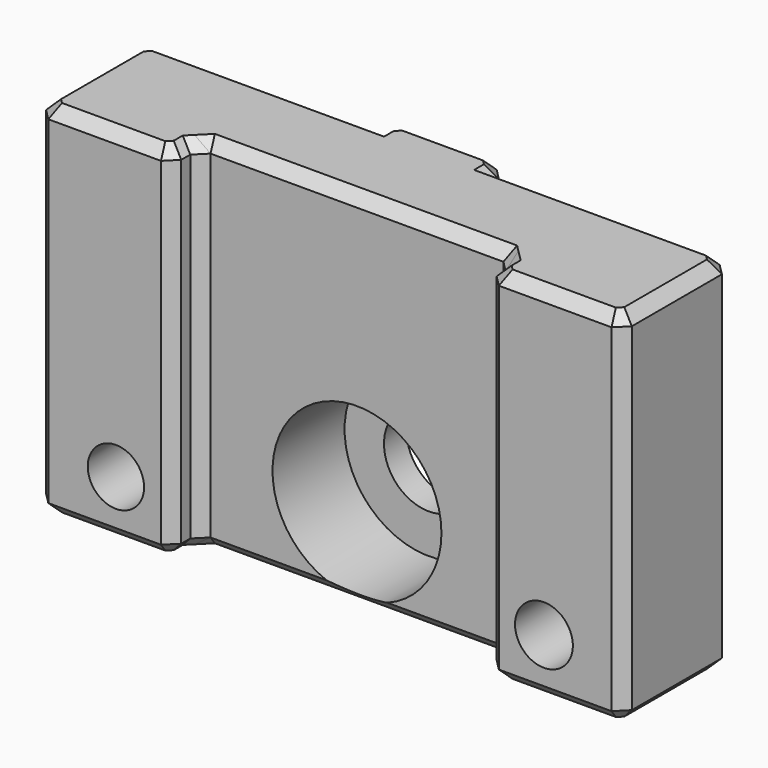
from build123d import *

# Parameters (mm, degrees)
F1_DEPTH      = 16
F3_R          = 1.25
F4_DEPTH      = 25
F5_R          = 2
F6_DEPTH      = 25
F5_R_2        = 3.75
F7_DEPTH      = 4
F8_SIZE       = 0.49999
F9_T1_DEPTH   = 3.278775627
F9_T3_DEPTH   = 7.571702988
F9_T5_DEPTH   = 3.278775627
F9_T7_DEPTH   = 6.571702988
F9_T9_DEPTH   = 7.571702988
F9_T11_DEPTH  = 3.278775627
F9_T13_DEPTH  = 3.278775627
F9_T15_DEPTH  = 3.278775627
F9_T17_DEPTH  = 7.571702988
F9_T19_DEPTH  = 3.278775627
F9_T24_DEPTH  = 12.571692988
F9_T29_DEPTH  = 2.821692988
F9_T34_DEPTH  = 3.278775627
F9_T39_DEPTH  = 3.278775627
F9_T44_DEPTH  = 2.821692988
F9_T49_DEPTH  = 3.071702988
F9_T54_DEPTH  = 12.571692988
F9_T59_DEPTH  = 3.278775627
F9_T65_DEPTH  = 15.571702988
F9_T71_DEPTH  = 3.278775627
F9_T77_DEPTH  = 3.071702988
F9_T82_DEPTH  = 12.571692988
F9_T87_DEPTH  = 2.821692988
F9_T92_DEPTH  = 3.278775627
F9_T97_DEPTH  = 3.278775627
F9_T102_DEPTH = 2.821692988
F9_T107_DEPTH = 3.071702988
F9_T112_DEPTH = 12.571692988
F9_T117_DEPTH = 3.278775627
F9_T123_DEPTH = 15.571702988
F9_T129_DEPTH = 3.278775627
F9_T135_DEPTH = 3.071702988


# Not quite as in the source:
# - a fillet or chamfer that OpenCascade refuses, or shapes differently, is made with other operations: its cross-section is extruded or revolved along the edge and cut away or added
# - a fillet or chamfer is up to 0.001 mm smaller than in the source, because OpenCascade refuses the exact size


with BuildPart() as f1:
    # F0 (on Top) → F1 (new body)
    with BuildSketch(Plane.XY):
        Polygon((-2.5, 3.4985319469), (-13, 3.4985319469), (-13, -2.5014680531), (-7, -2.5014680531), (-7, -1.0014680531), (7, -1.0014680531), (7, -2.5014680531), (13, -2.5014680531), (13, 3.4985319469), (2.5, 3.4985319469), (2.5, 4.2485319469), (-2.5, 4.2485319469), align=None)
    extrude(amount=F1_DEPTH)

    # F3 (on offset) → F4 (cut)
    with BuildSketch(Plane.XZ.offset(2.5014680531)):
        with Locations((-9.5, 2.5)):
            Circle(F3_R)
        with BuildLine():
            ThreePointArc((10.7833518404, 2.5), (9.5, 3.7833518404), (8.2166481596, 2.5))
            ThreePointArc((8.2166481596, 2.5), (9.5, 1.2166481596), (10.7833518404, 2.5))
        make_face()
    extrude(amount=-F4_DEPTH, mode=Mode.SUBTRACT)

    # F5 (on face) → F6 (cut)
    with BuildSketch(Plane.XZ.offset(1.0014680531)):
        with Locations((0, 4)):
            Circle(F5_R)
    extrude(amount=-F6_DEPTH, mode=Mode.SUBTRACT)

    # F5 (on face) → F7 (cut)
    with BuildSketch(Plane.XZ.offset(1.0014680531)):
        with Locations((0, 4)):
            Circle(F5_R_2)
        with Locations((0, 4)):
            Circle(F5_R, mode=Mode.SUBTRACT)
    extrude(amount=-F7_DEPTH, mode=Mode.SUBTRACT)

    # F8 (size 0.5 in the source; OpenCascade refuses exactly that, so slightly less here)
    f8_edges = [f1.edges().sort_by_distance(p)[0] for p in [
        (-2.5, 4.248532, 8),
        (2.5, 4.248532, 8),
        (13, 3.498532, 8),
        (-13, 3.498532, 8),
        (-13, -2.501468, 8),
        (7, -2.501468, 8),
        (13, -2.501468, 8),
        (-7, -2.501468, 8),
        (-7, -1.001468, 8),
        (7, -1.001468, 8),
    ]]
    chamfer(f8_edges, length=F8_SIZE)

    # F9: chamfer of 0.5 on 44 edges, made by hand

    # F9_s2 → F9_t1 (cut)
    with BuildSketch(Plane(origin=(3.5915117866, -3.5915117866, 0), x_dir=(0, 0, 1), z_dir=(0.7071067812, -0.7071067812, 0))):
        Polygon((15.5, -11.3126774998), (16, -10.8126774998), (16, -11.3126774998), align=None)
        Polygon((0, -10.8126774998), (0.5, -11.3126774998), (0, -11.3126774998), align=None)
    extrude(amount=F9_T1_DEPTH, mode=Mode.SUBTRACT)

    # F9_s4 → F9_t3 (cut)
    with BuildSketch(Plane.XZ.offset(-4.2843834409)):
        Polygon((12.5, 16), (13, 15.5), (13, 16), align=None)
        Polygon((-12.5, 16), (-13, 15.5), (-13, 16), align=None)
        Polygon((12.5, 0), (13, 0.5), (13, 0), align=None)
        Polygon((-12.5, 0), (-13, 0.5), (-13, 0), align=None)
    extrude(amount=F9_T3_DEPTH, mode=Mode.SUBTRACT)

    # F9_s6 → F9_t5 (cut)
    with BuildSketch(Plane(origin=(6.4084882134, 6.4084882134, 0), x_dir=(0, 0, 1), z_dir=(-0.7071067812, -0.7071067812, 0))):
        Polygon((16, -10.1076468592), (15.5, -10.6076468592), (16, -10.6076468592), align=None)
        Polygon((0, -10.1076468592), (0.5, -10.6076468592), (0, -10.6076468592), align=None)
    extrude(amount=F9_T5_DEPTH, mode=Mode.SUBTRACT)

    # F9_s8 → F9_t7 (cut)
    with BuildSketch(Plane.YZ.offset(-3.285851494)):
        Polygon((3.7485319469, 16), (4.2485319469, 15.5), (4.2485319469, 16), align=None)
        Polygon((3.7485319469, 0), (4.2485319469, 0.5), (4.2485319469, 0), align=None)
    extrude(amount=F9_T7_DEPTH, mode=Mode.SUBTRACT)

    # F9_s10 → F9_t9 (cut)
    with BuildSketch(Plane.YZ.offset(6.214148506)):
        Polygon((-2.0014680531, 16), (-2.5014680531, 15.5), (-2.5014680531, 16), align=None)
        Polygon((-2.0014680531, 0), (-2.5014680531, 0.5), (-2.5014680531, 0), align=None)
    extrude(amount=F9_T9_DEPTH, mode=Mode.SUBTRACT)

    # F9_s12 → F9_t11 (cut)
    with BuildSketch(Plane(origin=(5.9099562665, -5.9099562665, 0), x_dir=(0, 0, 1), z_dir=(-0.7071067812, 0.7071067812, 0))):
        Polygon((16, 4.0344887646), (15.5, 3.5344887646), (16, 3.5344887646), align=None)
        Polygon((0, 4.0344887646), (0.5, 3.5344887646), (0, 3.5344887646), align=None)
    extrude(amount=F9_T11_DEPTH, mode=Mode.SUBTRACT)

    # F9_s14 → F9_t13 (cut)
    with BuildSketch(Plane(origin=(-3.5915117866, -3.5915117866, 0), x_dir=(0, 0, 1), z_dir=(-0.7071067812, -0.7071067812, 0))):
        Polygon((16, 10.8126774998), (15.5, 11.3126774998), (16, 11.3126774998), align=None)
        Polygon((0, 10.8126774998), (0.5, 11.3126774998), (0, 11.3126774998), align=None)
    extrude(amount=F9_T13_DEPTH, mode=Mode.SUBTRACT)

    # F9_s16 → F9_t15 (cut)
    with BuildSketch(Plane(origin=(-6.4084882134, 6.4084882134, 0), x_dir=(0, 0, 1), z_dir=(0.7071067812, -0.7071067812, 0))):
        Polygon((16, 10.1076468592), (15.5, 10.6076468592), (16, 10.6076468592), align=None)
        Polygon((0, 10.1076468592), (0.5, 10.6076468592), (0, 10.6076468592), align=None)
    extrude(amount=F9_T15_DEPTH, mode=Mode.SUBTRACT)

    # F9_s18 → F9_t17 (cut)
    with BuildSketch(Plane.YZ.offset(-13.785851494)):
        Polygon((-2.0014680531, 16), (-2.5014680531, 15.5), (-2.5014680531, 16), align=None)
        Polygon((-2.0014680531, 0), (-2.5014680531, 0.5), (-2.5014680531, 0), align=None)
    extrude(amount=F9_T17_DEPTH, mode=Mode.SUBTRACT)

    # F9_s20 → F9_t19 (cut)
    with BuildSketch(Plane(origin=(-5.9099562665, -5.9099562665, 0), x_dir=(0, 0, 1), z_dir=(0.7071067812, 0.7071067812, 0))):
        Polygon((16, -4.0344887646), (15.5, -3.5344887646), (16, -3.5344887646), align=None)
        Polygon((0, -4.0344887646), (0.5, -3.5344887646), (0, -3.5344887646), align=None)
    extrude(amount=F9_T19_DEPTH, mode=Mode.SUBTRACT)


with BuildPart() as f9_tool22:
    # F9_s23 → F9_t24 (new body)
    with BuildSketch(Plane.YZ.offset(13.785851494)):
        Polygon((3.4985319469, 15.5), (2.9985319469, 16), (3.4985319469, 16), align=None)
    extrude(amount=-F9_T24_DEPTH)

    split(bisect_by=Plane(origin=(9, 0, 9), x_dir=(0, 1, 0), z_dir=(0.7071067812, 0, 0.7071067812)), keep=Keep.TOP)


with BuildPart() as f1_1:
    add(f1.part)

    # F9_t21: cut F9_tool22
    add(f9_tool22.part, mode=Mode.SUBTRACT)


with BuildPart() as f9_tool27:
    # F9_s28 → F9_t29 (new body)
    with BuildSketch(Plane.XZ.offset(-2.2126904529)):
        Polygon((2.5, 15.5), (2, 16), (2.5, 16), align=None)
    extrude(amount=-F9_T29_DEPTH)

    split(bisect_by=Plane(origin=(0, 9.4992659735, 9.4992659735), x_dir=(1, 0, 0), z_dir=(0, 0.7071067812, 0.7071067812)), keep=Keep.TOP)


with BuildPart() as f1_2:
    add(f1_1.part)

    # F9_t26: cut F9_tool27
    add(f9_tool27.part, mode=Mode.SUBTRACT)


with BuildPart() as f9_tool32:
    # F9_s33 → F9_t34 (new body)
    with BuildSketch(Plane(origin=(0.2849562665, -0.2849562665, 0), x_dir=(0, 0, 1), z_dir=(-0.7071067812, 0.7071067812, 0))):
        Polygon((16, 3.9183863832), (15.5, 4.4183863832), (16, 4.4183863832), align=None)
    extrude(amount=F9_T34_DEPTH)

    split(bisect_by=Plane.YZ.offset(2.5), keep=Keep.BOTTOM)


with BuildPart() as f1_3:
    add(f1_2.part)

    # F9_t31: cut F9_tool32
    add(f9_tool32.part, mode=Mode.SUBTRACT)


with BuildPart() as f9_tool37:
    # F9_s38 → F9_t39 (new body)
    with BuildSketch(Plane(origin=(2.0334882134, 2.0334882134, 0), x_dir=(0, 0, 1), z_dir=(-0.7071067812, -0.7071067812, 0))):
        Polygon((16, 3.9183863832), (15.5, 4.4183863832), (16, 4.4183863832), align=None)
    extrude(amount=F9_T39_DEPTH)

    split(bisect_by=Plane.YZ.offset(-2.5), keep=Keep.TOP)


with BuildPart() as f1_4:
    add(f1_3.part)

    # F9_t36: cut F9_tool37
    add(f9_tool37.part, mode=Mode.SUBTRACT)


with BuildPart() as f9_tool42:
    # F9_s43 → F9_t44 (new body)
    with BuildSketch(Plane.XZ.offset(-5.0343834409)):
        Polygon((-2, 16), (-2.5, 15.5), (-2.5, 16), align=None)
    extrude(amount=F9_T44_DEPTH)

    split(bisect_by=Plane(origin=(0, 9.4992659735, 9.4992659735), x_dir=(1, 0, 0), z_dir=(0, 0.7071067812, 0.7071067812)), keep=Keep.TOP)


with BuildPart() as f1_5:
    add(f1_4.part)

    # F9_t41: cut F9_tool42
    add(f9_tool42.part, mode=Mode.SUBTRACT)


with BuildPart() as f9_tool47:
    # F9_s48 → F9_t49 (new body)
    with BuildSketch(Plane.XZ.offset(0.2156165591)):
        Polygon((7.5, 16), (7, 15.5), (7, 16), align=None)
    extrude(amount=F9_T49_DEPTH)

    split(bisect_by=Plane(origin=(-4.1054420675, -4.1054420675, 5.8059718513), x_dir=(0.7071067812, -0.7071067812, 0), z_dir=(-0.5, -0.5, 0.7071067812)), keep=Keep.TOP)


with BuildPart() as f1_6:
    add(f1_5.part)

    # F9_t46: cut F9_tool47
    add(f9_tool47.part, mode=Mode.SUBTRACT)


with BuildPart() as f9_tool52:
    # F9_s53 → F9_t54 (new body)
    with BuildSketch(Plane.YZ.offset(-1.214158506)):
        Polygon((2.9985319469, 16), (3.4985319469, 15.5), (3.4985319469, 16), align=None)
    extrude(amount=-F9_T54_DEPTH)

    split(bisect_by=Plane(origin=(-9, 0, 9), x_dir=(0, 1, 0), z_dir=(-0.7071067812, 0, 0.7071067812)), keep=Keep.TOP)


with BuildPart() as f1_7:
    add(f1_6.part)

    # F9_t51: cut F9_tool52
    add(f9_tool52.part, mode=Mode.SUBTRACT)


with BuildPart() as f9_tool57:
    # F9_s58 → F9_t59 (new body)
    with BuildSketch(Plane(origin=(2.8415117866, -2.8415117866, 0), x_dir=(0, 0, 1), z_dir=(0.7071067812, -0.7071067812, 0))):
        Polygon((16, -4.3880562973), (15.5, -3.8880562973), (16, -3.8880562973), align=None)
    extrude(amount=F9_T59_DEPTH)

    split(bisect_by=Plane(origin=(0, -8.2507340265, 8.2507340265), x_dir=(1, 0, 0), z_dir=(0, -0.7071067812, 0.7071067812)), keep=Keep.TOP)

    split(bisect_by=Plane(origin=(-4.25, 0, 4.25), x_dir=(0, 1, 0), z_dir=(-0.7071067812, 0, 0.7071067812)), keep=Keep.TOP)


with BuildPart() as f1_8:
    add(f1_7.part)

    # F9_t56: cut F9_tool57
    add(f9_tool57.part, mode=Mode.SUBTRACT)


with BuildPart() as f9_tool63:
    # F9_s64 → F9_t65 (new body)
    with BuildSketch(Plane.YZ.offset(-7.785851494)):
        Polygon((-0.5014680531, 16), (-1.0014680531, 15.5), (-1.0014680531, 16), align=None)
    extrude(amount=F9_T65_DEPTH)

    split(bisect_by=Plane(origin=(-4.1054420675, -4.1054420675, 5.8059718513), x_dir=(0.7071067812, -0.7071067812, 0), z_dir=(-0.5, -0.5, 0.7071067812)), keep=Keep.TOP)

    split(bisect_by=Plane(origin=(4.1054420675, -4.1054420675, 5.8059718513), x_dir=(0.7071067812, 0.7071067812, 0), z_dir=(0.5, -0.5, 0.7071067812)), keep=Keep.TOP)


with BuildPart() as f1_9:
    add(f1_8.part)

    # F9_t62: cut F9_tool63
    add(f9_tool63.part, mode=Mode.SUBTRACT)


with BuildPart() as f9_tool69:
    # F9_s70 → F9_t71 (new body)
    with BuildSketch(Plane(origin=(-5.1599562665, -5.1599562665, 0), x_dir=(0, 0, 1), z_dir=(0.7071067812, 0.7071067812, 0))):
        Polygon((16, -4.3880562973), (15.5, -3.8880562973), (16, -3.8880562973), align=None)
    extrude(amount=F9_T71_DEPTH)

    split(bisect_by=Plane(origin=(0, -8.2507340265, 8.2507340265), x_dir=(1, 0, 0), z_dir=(0, -0.7071067812, 0.7071067812)), keep=Keep.TOP)

    split(bisect_by=Plane(origin=(4.25, 0, 4.25), x_dir=(0, 1, 0), z_dir=(0.7071067812, 0, 0.7071067812)), keep=Keep.TOP)


with BuildPart() as f1_10:
    add(f1_9.part)

    # F9_t68: cut F9_tool69
    add(f9_tool69.part, mode=Mode.SUBTRACT)


with BuildPart() as f9_tool75:
    # F9_s76 → F9_t77 (new body)
    with BuildSketch(Plane.XZ.offset(3.2873195471)):
        Polygon((-7.5, 16), (-7, 15.5), (-7, 16), align=None)
    extrude(amount=-F9_T77_DEPTH)

    split(bisect_by=Plane(origin=(4.1054420675, -4.1054420675, 5.8059718513), x_dir=(0.7071067812, 0.7071067812, 0), z_dir=(0.5, -0.5, 0.7071067812)), keep=Keep.TOP)


with BuildPart() as f1_11:
    add(f1_10.part)

    # F9_t74: cut F9_tool75
    add(f9_tool75.part, mode=Mode.SUBTRACT)


with BuildPart() as f9_tool80:
    # F9_s81 → F9_t82 (new body)
    with BuildSketch(Plane.YZ.offset(13.785851494)):
        Polygon((3.4985319469, 0.5), (2.9985319469, 0), (3.4985319469, 0), align=None)
    extrude(amount=-F9_T82_DEPTH)

    split(bisect_by=Plane(origin=(1, 0, -1), x_dir=(0, 1, 0), z_dir=(0.7071067812, 0, -0.7071067812)), keep=Keep.TOP)


with BuildPart() as f1_12:
    add(f1_11.part)

    # F9_t79: cut F9_tool80
    add(f9_tool80.part, mode=Mode.SUBTRACT)


with BuildPart() as f9_tool85:
    # F9_s86 → F9_t87 (new body)
    with BuildSketch(Plane.XZ.offset(-2.2126904529)):
        Polygon((2, 0), (2.5, 0.5), (2.5, 0), align=None)
    extrude(amount=-F9_T87_DEPTH)

    split(bisect_by=Plane(origin=(0, 1.4992659735, -1.4992659735), x_dir=(1, 0, 0), z_dir=(0, 0.7071067812, -0.7071067812)), keep=Keep.TOP)


with BuildPart() as f1_13:
    add(f1_12.part)

    # F9_t84: cut F9_tool85
    add(f9_tool85.part, mode=Mode.SUBTRACT)


with BuildPart() as f9_tool90:
    # F9_s91 → F9_t92 (new body)
    with BuildSketch(Plane(origin=(0.2849562665, -0.2849562665, 0), x_dir=(0, 0, 1), z_dir=(-0.7071067812, 0.7071067812, 0))):
        Polygon((0, 3.9183863832), (0.5, 4.4183863832), (0, 4.4183863832), align=None)
    extrude(amount=F9_T92_DEPTH)

    split(bisect_by=Plane.YZ.offset(2.5), keep=Keep.BOTTOM)


with BuildPart() as f1_14:
    add(f1_13.part)

    # F9_t89: cut F9_tool90
    add(f9_tool90.part, mode=Mode.SUBTRACT)


with BuildPart() as f9_tool95:
    # F9_s96 → F9_t97 (new body)
    with BuildSketch(Plane(origin=(2.0334882134, 2.0334882134, 0), x_dir=(0, 0, 1), z_dir=(-0.7071067812, -0.7071067812, 0))):
        Polygon((0, 3.9183863832), (0.5, 4.4183863832), (0, 4.4183863832), align=None)
    extrude(amount=F9_T97_DEPTH)

    split(bisect_by=Plane.YZ.offset(-2.5), keep=Keep.TOP)


with BuildPart() as f1_15:
    add(f1_14.part)

    # F9_t94: cut F9_tool95
    add(f9_tool95.part, mode=Mode.SUBTRACT)


with BuildPart() as f9_tool100:
    # F9_s101 → F9_t102 (new body)
    with BuildSketch(Plane.XZ.offset(-5.0343834409)):
        Polygon((-2, 0), (-2.5, 0.5), (-2.5, 0), align=None)
    extrude(amount=F9_T102_DEPTH)

    split(bisect_by=Plane(origin=(0, 1.4992659735, -1.4992659735), x_dir=(1, 0, 0), z_dir=(0, 0.7071067812, -0.7071067812)), keep=Keep.TOP)


with BuildPart() as f1_16:
    add(f1_15.part)

    # F9_t99: cut F9_tool100
    add(f9_tool100.part, mode=Mode.SUBTRACT)


with BuildPart() as f9_tool105:
    # F9_s106 → F9_t107 (new body)
    with BuildSketch(Plane.XZ.offset(0.2156165591)):
        Polygon((7.5, 0), (7, 0.5), (7, 0), align=None)
    extrude(amount=F9_T107_DEPTH)

    split(bisect_by=Plane(origin=(1.551412182, 1.551412182, 2.1940281487), x_dir=(0.7071067812, -0.7071067812, 0), z_dir=(-0.5, -0.5, -0.7071067812)), keep=Keep.TOP)


with BuildPart() as f1_17:
    add(f1_16.part)

    # F9_t104: cut F9_tool105
    add(f9_tool105.part, mode=Mode.SUBTRACT)


with BuildPart() as f9_tool110:
    # F9_s111 → F9_t112 (new body)
    with BuildSketch(Plane.YZ.offset(-1.214158506)):
        Polygon((2.9985319469, 0), (3.4985319469, 0.5), (3.4985319469, 0), align=None)
    extrude(amount=-F9_T112_DEPTH)

    split(bisect_by=Plane(origin=(-1, 0, -1), x_dir=(0, 1, 0), z_dir=(-0.7071067812, 0, -0.7071067812)), keep=Keep.TOP)


with BuildPart() as f1_18:
    add(f1_17.part)

    # F9_t109: cut F9_tool110
    add(f9_tool110.part, mode=Mode.SUBTRACT)


with BuildPart() as f9_tool115:
    # F9_s116 → F9_t117 (new body)
    with BuildSketch(Plane(origin=(2.8415117866, -2.8415117866, 0), x_dir=(0, 0, 1), z_dir=(0.7071067812, -0.7071067812, 0))):
        Polygon((0, -4.3880562973), (0.5, -3.8880562973), (0, -3.8880562973), align=None)
    extrude(amount=F9_T117_DEPTH)

    split(bisect_by=Plane(origin=(0, -0.2507340265, -0.2507340265), x_dir=(1, 0, 0), z_dir=(0, -0.7071067812, -0.7071067812)), keep=Keep.TOP)

    split(bisect_by=Plane(origin=(3.75, 0, 3.75), x_dir=(0, 1, 0), z_dir=(-0.7071067812, 0, -0.7071067812)), keep=Keep.TOP)


with BuildPart() as f1_19:
    add(f1_18.part)

    # F9_t114: cut F9_tool115
    add(f9_tool115.part, mode=Mode.SUBTRACT)


with BuildPart() as f9_tool121:
    # F9_s122 → F9_t123 (new body)
    with BuildSketch(Plane.YZ.offset(-7.785851494)):
        Polygon((-0.5014680531, 0), (-1.0014680531, 0.5), (-1.0014680531, 0), align=None)
    extrude(amount=F9_T123_DEPTH)

    split(bisect_by=Plane(origin=(1.551412182, 1.551412182, 2.1940281487), x_dir=(0.7071067812, -0.7071067812, 0), z_dir=(-0.5, -0.5, -0.7071067812)), keep=Keep.TOP)

    split(bisect_by=Plane(origin=(-1.551412182, 1.551412182, 2.1940281487), x_dir=(0.7071067812, 0.7071067812, 0), z_dir=(0.5, -0.5, -0.7071067812)), keep=Keep.TOP)


with BuildPart() as f1_20:
    add(f1_19.part)

    # F9_t120: cut F9_tool121
    add(f9_tool121.part, mode=Mode.SUBTRACT)


with BuildPart() as f9_tool127:
    # F9_s128 → F9_t129 (new body)
    with BuildSketch(Plane(origin=(-5.1599562665, -5.1599562665, 0), x_dir=(0, 0, 1), z_dir=(0.7071067812, 0.7071067812, 0))):
        Polygon((0, -4.3880562973), (0.5, -3.8880562973), (0, -3.8880562973), align=None)
    extrude(amount=F9_T129_DEPTH)

    split(bisect_by=Plane(origin=(0, -0.2507340265, -0.2507340265), x_dir=(1, 0, 0), z_dir=(0, -0.7071067812, -0.7071067812)), keep=Keep.TOP)

    split(bisect_by=Plane(origin=(-3.75, 0, 3.75), x_dir=(0, 1, 0), z_dir=(0.7071067812, 0, -0.7071067812)), keep=Keep.TOP)


with BuildPart() as f1_21:
    add(f1_20.part)

    # F9_t126: cut F9_tool127
    add(f9_tool127.part, mode=Mode.SUBTRACT)


with BuildPart() as f9_tool133:
    # F9_s134 → F9_t135 (new body)
    with BuildSketch(Plane.XZ.offset(3.2873195471)):
        Polygon((-7.5, 0), (-7, 0.5), (-7, 0), align=None)
    extrude(amount=-F9_T135_DEPTH)

    split(bisect_by=Plane(origin=(-1.551412182, 1.551412182, 2.1940281487), x_dir=(0.7071067812, 0.7071067812, 0), z_dir=(0.5, -0.5, -0.7071067812)), keep=Keep.TOP)


with BuildPart() as f1_22:
    add(f1_21.part)

    # F9_t132: cut F9_tool133
    add(f9_tool133.part, mode=Mode.SUBTRACT)


solid = f1_22.part
